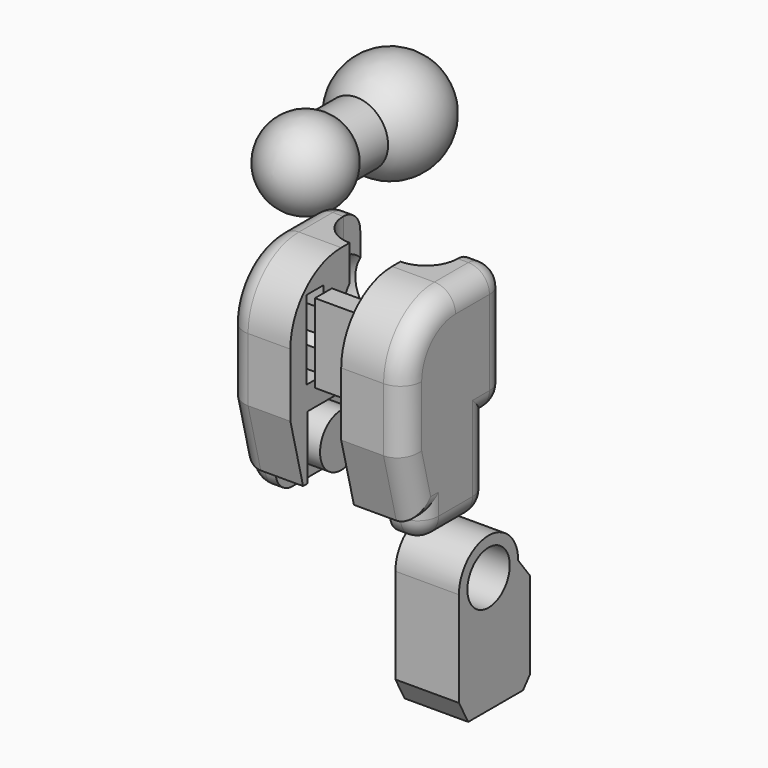
from build123d import *

# Parameters (mm, degrees)
F3_R           = 1.25
F4_DEPTH       = 3
F5_DEPTH       = 1.5
F9_DEPTH       = 2.5
F10_R          = 1.49999
F12_DEPTH      = 3.5
F13_DEPTH      = 0.5
F14_R          = 0.99999
F14_2_R        = 0.99999
F15_R          = 1.25
F16_DEPTH      = 3
F17_DEPTH      = 1
F18_T1_DEPTH   = 10.5
F18_T4_ANGLE   = 90
F18_2_T1_DEPTH = 10.5
F18_2_T4_ANGLE = 90


# Not quite as in the source:
# - a fillet or chamfer that OpenCascade refuses, or shapes differently, is made with other operations: its cross-section is extruded or revolved along the edge and cut away or added
# - a fillet or chamfer is up to 0.001 mm smaller than in the source, because OpenCascade refuses the exact size


with BuildPart() as f1:
    # F0 (on Right) → F1 (revolve)
    with BuildSketch(Plane.YZ):
        with BuildLine():
            Line((-5, 0), (2.5, 0))
            ThreePointArc((2.5, 0), (0.790569415, 2.3717082451), (-2, 1.5))
            Line((-2, 1.5), (-3.6771243445, 1.5))
            Line((-3.6771243445, 1.5), (-5, 1.5))
            Line((-5, 1.5), (-5, 0))
        make_face()
        with BuildLine():
            Line((-7, 0), (-5, 0))
            Line((-5, 0), (-5, 1.5))
            Line((-5, 1.5), (-3.6771243445, 1.5))
            ThreePointArc((-3.6771243445, 1.5), (-5.8228756555, 1.8228756555), (-7, 0))
        make_face()
    revolve(axis=Axis((0, -2.25, 0), (0, -1, 0)))


with BuildPart() as f4:
    # F3 (on offset) → F4 (new body)
    with BuildSketch(Plane.YZ.offset(8.3)):
        with BuildLine():
            Line((-10.2685662508, -0.4764611628), (-10.2685662508, 2.5235388372))
            Line((-10.2685662508, 2.5235388372), (-16.2685662508, 2.5235388372))
            Line((-16.2685662508, 2.5235388372), (-16.2685662508, -3.4764611628))
            Line((-16.2685662508, -3.4764611628), (-15.2685662508, -3.4764611628))
            Line((-15.2685662508, -3.4764611628), (-11.2685662508, -3.4764611628))
            Line((-11.2685662508, -3.4764611628), (-10.2685662508, -3.4764611628))
            Line((-10.2685662508, -3.4764611628), (-10.2685662508, -2.2085119704))
            ThreePointArc((-10.2685662508, -2.2085119704), (-12.2685662508, -2.2085119704), (-13.2685662508, -0.4764611628))
            Line((-13.2685662508, -0.4764611628), (-10.2685662508, -0.4764611628))
        make_face()
        Polygon((-14.3206530139, 1.389564241), (-14.3206530139, 0.389564241), (-13.8206530139, 0.1008891064), (-13.8206530139, -1.053811432), (-14.3206530139, -1.3424865666), (-14.3206530139, -2.3424865666), (-15.3206530139, -2.3424865666), (-15.3206530139, -1.3424865666), (-15.3206530139, 0.389564241), (-15.3206530139, 1.389564241), align=None, mode=Mode.SUBTRACT)
        Polygon((-11.2685662508, -3.4764611628), (-15.2685662508, -3.4764611628), (-15.2685662508, -6.4764611628), (-15.2685662508, -7.4764611628), (-11.2685662508, -7.4764611628), align=None)
        with Locations((-13.2685662508, -5.4764611628)):
            Circle(F3_R, mode=Mode.SUBTRACT)
        with BuildLine():
            Line((-10.2685662508, -2.2085119704), (-10.2685662508, -0.4764611628))
            Line((-10.2685662508, -0.4764611628), (-13.2685662508, -0.4764611628))
            ThreePointArc((-13.2685662508, -0.4764611628), (-12.2685662508, -2.2085119704), (-10.2685662508, -2.2085119704))
        make_face()
        with Locations((-13.2685662508, -5.4764611628)):
            Circle(F3_R)
        Polygon((-13.8206530139, 0.1008891064), (-14.3206530139, 0.389564241), (-14.3206530139, 1.389564241), (-15.3206530139, 1.389564241), (-15.3206530139, 0.389564241), (-15.3206530139, -1.3424865666), (-15.3206530139, -2.3424865666), (-14.3206530139, -2.3424865666), (-14.3206530139, -1.3424865666), (-13.8206530139, -1.053811432), align=None)
        Polygon((-15.2685662508, -3.4764611628), (-16.2685662508, -3.4764611628), (-15.5185662508, -6.4764611628), (-15.2685662508, -6.4764611628), align=None)
    extrude(amount=-F4_DEPTH)

    # F3 (on offset) → F5 (cut)
    with BuildSketch(Plane.YZ.offset(8.3)):
        Polygon((-11.2685662508, -3.4764611628), (-15.2685662508, -3.4764611628), (-15.2685662508, -6.4764611628), (-15.2685662508, -7.4764611628), (-11.2685662508, -7.4764611628), align=None)
        with Locations((-13.2685662508, -5.4764611628)):
            Circle(F3_R, mode=Mode.SUBTRACT)
        Polygon((-13.8206530139, 0.1008891064), (-14.3206530139, 0.389564241), (-14.3206530139, 1.389564241), (-15.3206530139, 1.389564241), (-15.3206530139, 0.389564241), (-15.3206530139, -1.3424865666), (-15.3206530139, -2.3424865666), (-14.3206530139, -2.3424865666), (-14.3206530139, -1.3424865666), (-13.8206530139, -1.053811432), align=None)
    extrude(amount=-F5_DEPTH, mode=Mode.SUBTRACT)

    # F3 (on offset) → F6 (revolve, cut)
    with BuildSketch(Plane.YZ.offset(8.3)):
        with BuildLine():
            Line((-10.2685662508, -2.2085119704), (-10.2685662508, -0.4764611628))
            Line((-10.2685662508, -0.4764611628), (-13.2685662508, -0.4764611628))
            ThreePointArc((-13.2685662508, -0.4764611628), (-12.2685662508, -2.2085119704), (-10.2685662508, -2.2085119704))
        make_face()
    revolve(axis=Axis((8.3, -11.2685662508, -0.4764611628), (0, -1, 0)), mode=Mode.SUBTRACT)

    # F8 (on face) → F9 (cut)
    with BuildSketch(Plane(origin=(0, -10.2685662508, 0), x_dir=(-1, 0, 0), z_dir=(0, 1, 0))):
        with BuildLine():
            ThreePointArc((-8.3, 1.2555896448), (-7.4339745962, 1.0235388372), (-6.8, 0.389564241))
            Line((-6.8, 0.389564241), (-6.8, 2.5235388372))
            Line((-6.8, 2.5235388372), (-8.3, 2.5235388372))
            Line((-8.3, 2.5235388372), (-8.3, 1.2555896448))
        make_face()
        with BuildLine():
            Line((-8.3, 0.389564241), (-6.8, 0.389564241))
            ThreePointArc((-6.8, 0.389564241), (-7.4339745962, 1.0235388372), (-8.3, 1.2555896448))
            Line((-8.3, 1.2555896448), (-8.3, 0.389564241))
        make_face()
    extrude(amount=-F9_DEPTH, mode=Mode.SUBTRACT)

    # F10 (radius 1.5 in the source; OpenCascade refuses exactly that, so slightly less here)
    f10_edges = [f4.edges().sort_by_distance(p)[0] for p in [
        (6.8, -12.768566, 1.456552),
    ]]
    fillet(f10_edges, radius=F10_R)


with BuildPart() as f11_1:
    # F11: instance of F4
    add(f4.part.mirror(Plane.YZ.offset(9.5)))

    # F12 (add): a face of the model
    f12_faces = [f11_1.faces().sort_by_distance(p)[0] for p in [
        (12.2, -14.7018230175, -0.4764611628),
    ]]
    extrude(f12_faces, amount=F12_DEPTH)

    # F14#2 (radius 1 in the source; OpenCascade refuses exactly that, so slightly less here)
    f14_2_edges = [f11_1.edges().sort_by_distance(p)[0] for p in [
        (13.7, -15.268566, -6.976461),
        (13.7, -13.268566, -7.476461),
        (13.7, -11.268566, -5.476461),
        (13.7, -10.768566, -3.476461),
        (13.7, -10.268566, -0.476461),
        (13.7, -13.268566, 2.523539),
        (13.7, -16.268566, -0.476461),
        (13.7, -15.893566, -4.976461),
        (13.7, -15.393566, -6.476461),
        (12.95, -10.268566, 2.523539),
        (12.2, -10.268566, -3.476461),
        (12.95, -11.268566, -7.476461),
        (12.95, -15.268566, -7.476461),
    ]]
    fillet(f14_2_edges, radius=F14_2_R)

    # F18#2: fillet of radius 3 on 1 edges, made by hand

    # F18_2_s2 → F18_2_t1 (cut)
    with BuildSketch(Plane.YZ.offset(3.2)):
        with BuildLine():
            ThreePointArc((-13.2685662508, 2.5235388372), (-15.3898865944, 1.6448591808), (-16.2685662508, -0.4764611628))
            Line((-16.2685662508, -0.4764611628), (-16.2685662508, 2.5235388372))
            Line((-16.2685662508, 2.5235388372), (-13.2685662508, 2.5235388372))
        make_face()
    extrude(amount=F18_2_T1_DEPTH, mode=Mode.SUBTRACT)

    # F18_2_s3 → F18_2_t4 (revolve, cut)
    with BuildSketch(Plane.XZ.offset(13.2685662508)):
        with BuildLine():
            ThreePointArc((13.7, 1.5235488372), (13.4071097101, 2.2306485473), (12.70001, 2.5235388372))
            Line((12.70001, 2.5235388372), (13.7, 2.5235388372))
            Line((13.7, 2.5235388372), (13.7, 1.5235488372))
        make_face()
    revolve(axis=Axis((13.7, -13.2685662508, -0.4764611628), (1, 0, 0)), revolution_arc=F18_2_T4_ANGLE, mode=Mode.SUBTRACT)


with BuildPart() as f4_1:
    add(f4.part)

    # F13 (cut): a face of the model
    f13_faces = [f4_1.faces().sort_by_distance(p)[0] for p in [
        (6.8, -14.7018230175, -0.4764611628),
    ]]
    extrude(f13_faces, amount=-F13_DEPTH, mode=Mode.SUBTRACT)

    # F14 (radius 1 in the source; OpenCascade refuses exactly that, so slightly less here)
    f14_edges = [f4_1.edges().sort_by_distance(p)[0] for p in [
        (5.3, -15.268566, -6.976461),
        (5.3, -13.268566, -7.476461),
        (5.3, -11.268566, -5.476461),
        (5.3, -10.768566, -3.476461),
        (5.3, -10.268566, -0.476461),
        (5.3, -13.268566, 2.523539),
        (5.3, -16.268566, -0.476461),
        (5.3, -15.893566, -4.976461),
        (5.3, -15.393566, -6.476461),
        (6.05, -10.268566, 2.523539),
        (6.8, -10.268566, -3.476461),
        (6.05, -15.268566, -7.476461),
        (6.05, -11.268566, -7.476461),
    ]]
    fillet(f14_edges, radius=F14_R)

    # F18: fillet of radius 3 on 1 edges, made by hand

    # F18_s2 → F18_t1 (cut)
    with BuildSketch(Plane.YZ.offset(5.3)):
        with BuildLine():
            ThreePointArc((-13.2685662508, 2.5235388372), (-15.3898865944, 1.6448591808), (-16.2685662508, -0.4764611628))
            Line((-16.2685662508, -0.4764611628), (-16.2685662508, 2.5235388372))
            Line((-16.2685662508, 2.5235388372), (-13.2685662508, 2.5235388372))
        make_face()
    extrude(amount=F18_T1_DEPTH, mode=Mode.SUBTRACT)

    # F18_s3 → F18_t4 (revolve, cut)
    with BuildSketch(Plane.XY.offset(-0.4764611628)):
        with BuildLine():
            ThreePointArc((5.3, -15.2685762508), (5.5928902899, -15.9756759609), (6.29999, -16.2685662508))
            Line((6.29999, -16.2685662508), (5.3, -16.2685662508))
            Line((5.3, -16.2685662508), (5.3, -15.2685762508))
        make_face()
    revolve(axis=Axis((5.3, -13.2685662508, -0.4764611628), (-1, 0, 0)), revolution_arc=F18_T4_ANGLE, mode=Mode.SUBTRACT)


with BuildPart() as f16:
    # F15 (on offset) → F16 (new body)
    with BuildSketch(Plane.YZ.offset(9.5)):
        with BuildLine():
            ThreePointArc((-11.5690167919, -11.2316595539), (-9.8190167919, -12.9816595539), (-8.0690167919, -11.2316595539))
            ThreePointArc((-8.0690167919, -11.2316595539), (-9.8190167919, -9.4816595539), (-11.5690167919, -11.2316595539))
        make_face()
        with Locations((-9.8190167919, -11.2316595539)):
            Circle(F15_R, mode=Mode.SUBTRACT)
        with BuildLine():
            Line((-7.3671324644, -12.1526874641), (-8.0690167919, -11.2316595539))
            ThreePointArc((-8.0690167919, -11.2316595539), (-9.8190167919, -12.9816595539), (-11.5690167919, -11.2316595539))
            Line((-11.5690167919, -11.2316595539), (-11.5690167919, -14.7316595539))
            Line((-11.5690167919, -14.7316595539), (-11.0185509548, -15.7451722771))
            Line((-11.0185509548, -15.7451722771), (-7.7812108211, -15.7451722771))
            Line((-7.7812108211, -15.7451722771), (-7.3671324644, -15.2384159155))
            Line((-7.3671324644, -15.2384159155), (-7.3671324644, -12.1526874641))
        make_face()
    extrude(amount=F16_DEPTH)

    # F17 (add): faces of the model
    f17_faces = [f16.faces().sort_by_distance(p)[0] for p in [
        (11, -9.3998808879, -15.7451722771),
        (11, -11.2937838733, -15.2384159155),
        (11, -7.5741716428, -15.4917940963),
    ]]
    extrude(f17_faces, amount=F17_DEPTH, dir=(0, 0, -1))


solid = Compound([f1.part, f11_1.part, f4_1.part, f16.part])
